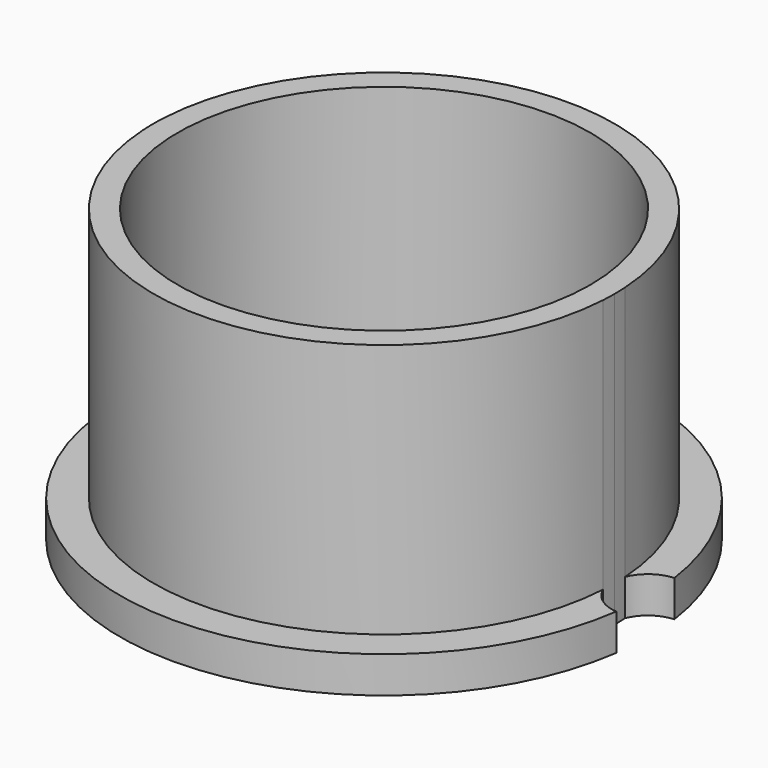
from build123d import *

# Parameters (mm, degrees)
F0_R     = 17
F1_DEPTH = 3
F2_DEPTH = 24


with BuildPart() as f1:
    # F0 (on Top) → F1 (new body)
    with BuildSketch(Plane.XY):
        with BuildLine():
            ThreePointArc((18.966954023, 1.1201138736), (19.9859901049, 2.4265755892), (21.5431034483, 2.9928571327))
            ThreePointArc((21.5431034483, 2.9928571327), (0, 21.75), (-21.5431034483, 2.9928571327))
            ThreePointArc((-21.5431034483, 2.9928571327), (-19.9859901049, 2.4265755892), (-18.966954023, 1.1201138736))
            ThreePointArc((-18.966954023, 1.1201138736), (0, 19), (18.966954023, 1.1201138736))
        make_face()
        with BuildLine():
            ThreePointArc((-21.5431034483, -2.9928571327), (0, -21.75), (21.5431034483, -2.9928571327))
            ThreePointArc((21.5431034483, -2.9928571327), (19.9859901049, -2.4265755892), (18.966954023, -1.1201138736))
            ThreePointArc((18.966954023, -1.1201138736), (0, -19), (-18.966954023, -1.1201138736))
            ThreePointArc((-18.966954023, -1.1201138736), (-19.9859901049, -2.4265755892), (-21.5431034483, -2.9928571327))
        make_face()
        with BuildLine():
            ThreePointArc((18.966954023, -1.1201138736), (18.75, 0), (18.966954023, 1.1201138736))
            ThreePointArc((18.966954023, 1.1201138736), (0, 19), (-18.966954023, 1.1201138736))
            ThreePointArc((-18.966954023, 1.1201138736), (-18.8047378783, 0.5704656295), (-18.75, 0))
            ThreePointArc((-18.75, 0), (-18.8047378783, -0.5704656295), (-18.966954023, -1.1201138736))
            ThreePointArc((-18.966954023, -1.1201138736), (0, -19), (18.966954023, -1.1201138736))
        make_face()
        Circle(F0_R, mode=Mode.SUBTRACT)
    extrude(amount=F1_DEPTH)

    # F0 (on Top) → F2 (join)
    with BuildSketch(Plane.XY):
        with BuildLine():
            ThreePointArc((18.966954023, -1.1201138736), (18.75, 0), (18.966954023, 1.1201138736))
            ThreePointArc((18.966954023, 1.1201138736), (0, 19), (-18.966954023, 1.1201138736))
            ThreePointArc((-18.966954023, 1.1201138736), (-18.8047378783, 0.5704656295), (-18.75, 0))
            ThreePointArc((-18.75, 0), (-18.8047378783, -0.5704656295), (-18.966954023, -1.1201138736))
            ThreePointArc((-18.966954023, -1.1201138736), (0, -19), (18.966954023, -1.1201138736))
        make_face()
        Circle(F0_R, mode=Mode.SUBTRACT)
        with BuildLine():
            ThreePointArc((-18.75, 0), (-18.8047378783, 0.5704656295), (-18.966954023, 1.1201138736))
            ThreePointArc((-18.966954023, 1.1201138736), (-19, 0), (-18.966954023, -1.1201138736))
            ThreePointArc((-18.966954023, -1.1201138736), (-18.8047378783, -0.5704656295), (-18.75, 0))
        make_face()
        with BuildLine():
            ThreePointArc((19, 0), (18.9917367089, 0.5603006172), (18.966954023, 1.1201138736))
            ThreePointArc((18.966954023, 1.1201138736), (18.75, 0), (18.966954023, -1.1201138736))
            ThreePointArc((18.966954023, -1.1201138736), (18.9917367089, -0.5603006172), (19, 0))
        make_face()
    extrude(amount=F2_DEPTH)


solid = f1.part
